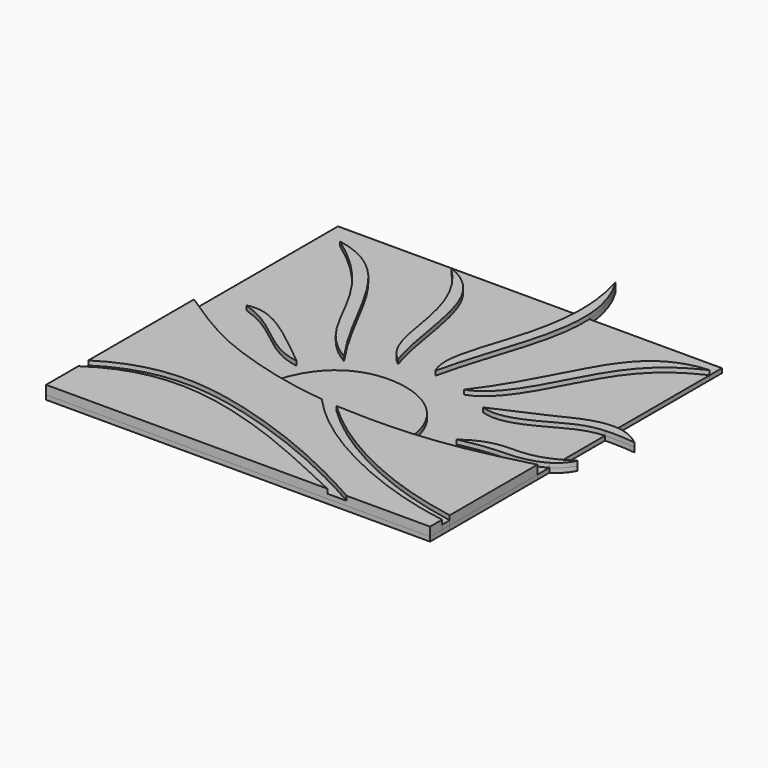
from build123d import *

# Parameters (mm, degrees)
F1_DEPTH = 0.8
F2_DEPTH = 0.8
F4_DEPTH = 0.8


# Not quite as in the source:
# - the dataset's text gives a spline's control points without its knots; the knots are read off the source's solid


with BuildPart() as f1:
    # F0 (on Top) → F1 (new body)
    with BuildSketch(Plane.XY):
        with BuildLine():
            Line((34.9730342203, 35.0006110966), (10.9699166685, 35.0006110966))
            add(Edge.make_bspline(
                [(10.9699166685, 35.0006110966), (11.4434143594, 26.4683997801), (6.9927337903, 17.8281453772), (4.7980677336, 7.8657846898)],
                knots=[10.4639255088, 10.4639255088, 10.4639255088, 10.4639255088, 37.2667273863, 37.2667273863, 37.2667273863, 37.2667273863], degree=3))
            add(Edge.make_bspline(
                [(9.1649998173, 35.0006110966), (8.9947581749, 22.5710061914), (1.9450564413, 13.7213998068), (4.7980677336, 7.8657846898)],
                knots=[7.4607386128, 7.4607386128, 7.4607386128, 7.4607386128, 37.2667273863, 37.2667273863, 37.2667273863, 37.2667273863], degree=3))
            Line((9.1649998173, 35.0006110966), (-34.5254550172, 35.0006110966))
            Line((-34.5254550172, 35.0006110966), (-34.5254550172, 2.4173662354))
            add(Edge.make_bspline(
                [(-34.5254550172, 2.4173662354), (-27.0376804173, -2.6116999925), (-21.9956358256, -5.211225175), (-13.8138692011, -7.7319000425), (-11.0227311637, -8.421960214)],
                knots=[0, 0, 0, 0, 0.5006994626, 0.7376571396, 0.7376571396, 0.7376571396, 0.7376571396], degree=3))
            add(Edge.make_bspline(
                [(-11.0227311637, -8.421960214), (-8.8453157151, -0.8208052436), (1.8576873576, 4.9563290965), (14.2170952187, -2.2695153177), (14.8043119806, -10.429123426)],
                knots=[0, 0, 0, 0, 0.4927942215, 1, 1, 1, 1], degree=3))
            add(Edge.make_bspline(
                [(14.8043119806, -10.429123426), (16.5213615363, -10.3106762034), (23.4560587989, -9.6183687732), (30.1043070095, -8.0231877273), (34.9773075939, -6.7529535132)],
                knots=[0.3679463332, 0.3679463332, 0.3679463332, 0.3679463332, 0.5212374468, 1, 1, 1, 1], degree=3))
            Line((34.9773075939, -6.7529535132), (34.9770299958, -4.040644467))
            add(Edge.make_bspline(
                [(20.261824131, -6.674728822), (25.9323026985, -5.3960913792), (28.2483273712, -6.1310401757), (33.4074649083, -4.9876865132), (34.9770299958, -4.040644467)],
                knots=[0, 0, 0, 0, 0.514073902, 0.7971639338, 0.7971639338, 0.7971639338, 0.7971639338], degree=3))
            add(Edge.make_bspline(
                [(20.261824131, -6.674728822), (24.2642636854, -3.7840772049), (28.8724834606, -4.3450209461), (32.8278065722, -3.6447079653), (34.976883526, -2.609541392)],
                knots=[0, 0, 0, 0, 0.5118221944, 0.8647946005, 0.8647946005, 0.8647946005, 0.8647946005], degree=3))
            Line((34.976883526, -2.609541392), (34.9757434519, 8.5297036957))
            add(Edge.make_bspline(
                [(17.0930270106, 3.331998596), (21.0957173258, 1.9421754405), (28.3670720206, 6.719546536), (32.5488536668, 8.3655302085), (34.9757434519, 8.5297036957)],
                knots=[0, 0, 0, 0, 0.5070444455, 0.8166137967, 0.8166137967, 0.8166137967, 0.8166137967], degree=3))
            add(Edge.make_bspline(
                [(17.0930270106, 3.331998596), (24.4312938303, 6.6675744019), (25.142738508, 6.7759703545), (32.0404376887, 10.3392415102), (34.9755569111, 10.3523255806)],
                knots=[0, 0, 0, 0, 0.4853131484, 0.8039573304, 0.8039573304, 0.8039573304, 0.8039573304], degree=3))
            Line((34.9755569111, 10.3523255806), (34.9733161214, 32.246258361))
            Line((34.9733161214, 32.246258361), (34.9730342203, 35.0006110966))
        make_face()
        with BuildLine():
            add(Edge.make_bspline(
                [(-28.5548307002, 6.8228477612), (-21.2621595711, 4.5322012156), (-18.9715120941, -1.030798303), (-12.3800588772, -2.0125040319)],
                knots=[0, 0, 0, 0, 18.4305910061, 18.4305910061, 18.4305910061, 18.4305910061], degree=3))
            add(Edge.make_bspline(
                [(-28.5548307002, 6.8228477612), (-24.1137798876, 8.0850413069), (-18.9715120941, 3.1765124295), (-12.3800588772, -2.0125040319)],
                knots=[0, 0, 0, 0, 18.4305910061, 18.4305910061, 18.4305910061, 18.4305910061], degree=3))
        make_face(mode=Mode.SUBTRACT)
        with BuildLine():
            add(Edge.make_bspline(
                [(-30.4424781352, 30.3799584508), (-14.8932319134, 19.365908578), (-18.1915573776, 9.1764414683), (-8.0609880388, 3.2865752)],
                knots=[0, 0, 0, 0, 35.1423180071, 35.1423180071, 35.1423180071, 35.1423180071], degree=3))
            add(Edge.make_bspline(
                [(-30.4424781352, 30.3799584508), (-18.3093566447, 28.1418096274), (-16.7779885232, 15.8319901675), (-8.0609880388, 3.2865752)],
                knots=[0, 0, 0, 0, 35.1423180071, 35.1423180071, 35.1423180071, 35.1423180071], degree=3))
        make_face(mode=Mode.SUBTRACT)
        with BuildLine():
            add(Edge.make_bspline(
                [(-13.0653008819, 33.8075049222), (-3.1436614227, 24.1144448519), (-7.886134088, 12.1958628297), (-1.5212370781, 7.3285889812)],
                knots=[0, 0, 0, 0, 28.885955039, 28.885955039, 28.885955039, 28.885955039], degree=3))
            add(Edge.make_bspline(
                [(-13.0653008819, 33.8075049222), (-3.081260249, 29.9177337438), (-5.0780908205, 18.31115596), (-1.5212370781, 7.3285889812)],
                knots=[0, 0, 0, 0, 28.885955039, 28.885955039, 28.885955039, 28.885955039], degree=3))
        make_face(mode=Mode.SUBTRACT)
        with BuildLine():
            add(Edge.make_bspline(
                [(34.9733161214, 32.246258361), (26.694862172, 31.7585282028), (20.0014700507, 20.5728578228), (15.3970348817, 10.8755724271), (11.565268971, 5.9131206945)],
                knots=[0, 0, 0, 0, 0.5086442243, 1, 1, 1, 1], degree=3))
            add(Edge.make_bspline(
                [(34.9733161214, 32.246258361), (28.0495304614, 29.0197413415), (22.3665736308, 20.9948728696), (16.2112628167, 7.3571462772), (11.565268971, 5.9131206945)],
                knots=[0, 0, 0, 0, 0.5063383757, 1, 1, 1, 1], degree=3))
        make_face(mode=Mode.SUBTRACT)
        with BuildLine():
            add(Edge.make_bspline(
                [(-34.5254550172, 2.4173662354), (-27.0376804173, -2.6116999925), (-21.9956358256, -5.211225175), (-13.8138692011, -7.7319000425), (-11.0227311637, -8.421960214)],
                knots=[0, 0, 0, 0, 0.5006994626, 0.7376571396, 0.7376571396, 0.7376571396, 0.7376571396], degree=3))
            Line((-34.5254550172, 2.4173662354), (-34.5254550172, -21.5029727188))
            add(Edge.make_bspline(
                [(-34.5254550172, -21.5029727188), (-25.4725657698, -15.6213664106), (-6.7297761633, -18.0960890657), (10.8723963711, -25.9276739276), (19.8863351902, -31.0484187179)],
                knots=[0, 0, 0, 0, 0.4889236203, 1, 1, 1, 1], degree=3))
            Line((19.8863351902, -31.0484187179), (34.9797941745, -31.0484187179))
            Line((34.9797941745, -31.0484187179), (34.9795152363, -28.32301612))
            add(Edge.make_bspline(
                [(-1.3718163174, -10.1225785816), (3.8546116383, -15.8494096152), (16.1560983213, -23.3323485383), (28.3092996314, -27.2113128984), (34.9795152363, -28.32301612)],
                knots=[0, 0, 0, 0, 0.5146424098, 1, 1, 1, 1], degree=3))
            add(Edge.make_bspline(
                [(-11.0227311637, -8.421960214), (-7.9325795984, -9.1859462621), (-4.6427454411, -9.8032650716), (-1.3718163174, -10.1225785816)],
                knots=[0.7376571396, 0.7376571396, 0.7376571396, 0.7376571396, 1, 1, 1, 1], degree=3))
        make_face()
        with BuildLine():
            add(Edge.make_bspline(
                [(-34.5254550172, -23.7555388327), (-26.0445526205, -17.8952354176), (-8.0264611969, -19.3880719353), (8.0517873689, -27.1572651783), (16.3802922747, -31.0484187179)],
                knots=[0, 0, 0, 0, 0.4951755821, 1, 1, 1, 1], degree=3))
            Line((-34.5254550172, -23.7555388327), (-34.5254550172, -31.0484187179))
            Line((-34.5254550172, -31.0484187179), (16.3802922747, -31.0484187179))
        make_face()
        with BuildLine():
            add(Edge.make_bspline(
                [(14.8043119806, -10.429123426), (16.5213615363, -10.3106762034), (23.4560587989, -9.6183687732), (30.1043070095, -8.0231877273), (34.9773075939, -6.7529535132)],
                knots=[0.3679463332, 0.3679463332, 0.3679463332, 0.3679463332, 0.5212374468, 1, 1, 1, 1], degree=3))
            add(Edge.make_bspline(
                [(1.5781647526, -10.4776900262), (6.3586774053, -10.7127967269), (10.6828591895, -10.7134335873), (14.8043119806, -10.429123426)],
                knots=[0, 0, 0, 0, 0.3679463332, 0.3679463332, 0.3679463332, 0.3679463332], degree=3))
            add(Edge.make_bspline(
                [(1.5781647526, -10.4776900262), (6.0786014384, -14.8114432857), (16.8554999855, -21.6973110945), (28.304374887, -25.3758922346), (34.9793388523, -26.599633516)],
                knots=[0, 0, 0, 0, 0.4979262009, 1, 1, 1, 1], degree=3))
            Line((34.9793388523, -26.599633516), (34.9773075939, -6.7529535132))
        make_face()
        with BuildLine():
            add(Edge.make_bspline(
                [(-11.0227311637, -8.421960214), (-8.8453157151, -0.8208052436), (1.8576873576, 4.9563290965), (14.2170952187, -2.2695153177), (14.8043119806, -10.429123426)],
                knots=[0, 0, 0, 0, 0.4927942215, 1, 1, 1, 1], degree=3))
            add(Edge.make_bspline(
                [(-11.0227311637, -8.421960214), (-7.9325795984, -9.1859462621), (-4.6427454411, -9.8032650716), (-1.3718163174, -10.1225785816)],
                knots=[0.7376571396, 0.7376571396, 0.7376571396, 0.7376571396, 1, 1, 1, 1], degree=3))
            add(Edge.make_bspline(
                [(-1.3718163174, -10.1225785816), (3.8546116383, -15.8494096152), (16.1560983213, -23.3323485383), (28.3092996314, -27.2113128984), (34.9795152363, -28.32301612)],
                knots=[0, 0, 0, 0, 0.5146424098, 1, 1, 1, 1], degree=3))
            Line((34.9795152363, -28.32301612), (34.9793388523, -26.599633516))
            add(Edge.make_bspline(
                [(1.5781647526, -10.4776900262), (6.0786014384, -14.8114432857), (16.8554999855, -21.6973110945), (28.304374887, -25.3758922346), (34.9793388523, -26.599633516)],
                knots=[0, 0, 0, 0, 0.4979262009, 1, 1, 1, 1], degree=3))
            add(Edge.make_bspline(
                [(1.5781647526, -10.4776900262), (6.3586774053, -10.7127967269), (10.6828591895, -10.7134335873), (14.8043119806, -10.429123426)],
                knots=[0, 0, 0, 0, 0.3679463332, 0.3679463332, 0.3679463332, 0.3679463332], degree=3))
        make_face()
        with BuildLine():
            add(Edge.make_bspline(
                [(-34.5254550172, -21.5029727188), (-25.4725657698, -15.6213664106), (-6.7297761633, -18.0960890657), (10.8723963711, -25.9276739276), (19.8863351902, -31.0484187179)],
                knots=[0, 0, 0, 0, 0.4889236203, 1, 1, 1, 1], degree=3))
            Line((-34.5254550172, -21.5029727188), (-34.5254550172, -23.7555388327))
            add(Edge.make_bspline(
                [(-34.5254550172, -23.7555388327), (-26.0445526205, -17.8952354176), (-8.0264611969, -19.3880719353), (8.0517873689, -27.1572651783), (16.3802922747, -31.0484187179)],
                knots=[0, 0, 0, 0, 0.4951755821, 1, 1, 1, 1], degree=3))
            Line((16.3802922747, -31.0484187179), (19.8863351902, -31.0484187179))
        make_face()
        with BuildLine():
            add(Edge.make_bspline(
                [(-30.4424781352, 30.3799584508), (-18.3093566447, 28.1418096274), (-16.7779885232, 15.8319901675), (-8.0609880388, 3.2865752)],
                knots=[0, 0, 0, 0, 35.1423180071, 35.1423180071, 35.1423180071, 35.1423180071], degree=3))
            add(Edge.make_bspline(
                [(-30.4424781352, 30.3799584508), (-14.8932319134, 19.365908578), (-18.1915573776, 9.1764414683), (-8.0609880388, 3.2865752)],
                knots=[0, 0, 0, 0, 35.1423180071, 35.1423180071, 35.1423180071, 35.1423180071], degree=3))
        make_face()
        with BuildLine():
            add(Edge.make_bspline(
                [(34.9733161214, 32.246258361), (28.0495304614, 29.0197413415), (22.3665736308, 20.9948728696), (16.2112628167, 7.3571462772), (11.565268971, 5.9131206945)],
                knots=[0, 0, 0, 0, 0.5063383757, 1, 1, 1, 1], degree=3))
            add(Edge.make_bspline(
                [(34.9733161214, 32.246258361), (26.694862172, 31.7585282028), (20.0014700507, 20.5728578228), (15.3970348817, 10.8755724271), (11.565268971, 5.9131206945)],
                knots=[0, 0, 0, 0, 0.5086442243, 1, 1, 1, 1], degree=3))
        make_face()
        with BuildLine():
            add(Edge.make_bspline(
                [(7.7365408652, 45.0164824724), (9.8496850647, 41.6461653484), (10.7850611974, 38.3316219383), (10.9699166685, 35.0006110966)],
                knots=[0, 0, 0, 0, 10.4639255088, 10.4639255088, 10.4639255088, 10.4639255088], degree=3))
            add(Edge.make_bspline(
                [(7.7365408652, 45.0164824724), (8.8191927924, 41.4474264531), (9.2076130117, 38.1118661522), (9.1649998173, 35.0006110966)],
                knots=[0, 0, 0, 0, 7.4607386128, 7.4607386128, 7.4607386128, 7.4607386128], degree=3))
            add(Edge.make_bspline(
                [(9.1649998173, 35.0006110966), (8.9947581749, 22.5710061914), (1.9450564413, 13.7213998068), (4.7980677336, 7.8657846898)],
                knots=[7.4607386128, 7.4607386128, 7.4607386128, 7.4607386128, 37.2667273863, 37.2667273863, 37.2667273863, 37.2667273863], degree=3))
            add(Edge.make_bspline(
                [(10.9699166685, 35.0006110966), (11.4434143594, 26.4683997801), (6.9927337903, 17.8281453772), (4.7980677336, 7.8657846898)],
                knots=[10.4639255088, 10.4639255088, 10.4639255088, 10.4639255088, 37.2667273863, 37.2667273863, 37.2667273863, 37.2667273863], degree=3))
        make_face()
        with BuildLine():
            add(Edge.make_bspline(
                [(-13.0653008819, 33.8075049222), (-3.081260249, 29.9177337438), (-5.0780908205, 18.31115596), (-1.5212370781, 7.3285889812)],
                knots=[0, 0, 0, 0, 28.885955039, 28.885955039, 28.885955039, 28.885955039], degree=3))
            add(Edge.make_bspline(
                [(-13.0653008819, 33.8075049222), (-3.1436614227, 24.1144448519), (-7.886134088, 12.1958628297), (-1.5212370781, 7.3285889812)],
                knots=[0, 0, 0, 0, 28.885955039, 28.885955039, 28.885955039, 28.885955039], degree=3))
        make_face()
        with BuildLine():
            add(Edge.make_bspline(
                [(34.9755569111, 10.3523255806), (36.7813598733, 10.3603754249), (38.6633412268, 9.8387998398), (40.4420569539, 8.3353621885)],
                knots=[0.8039573304, 0.8039573304, 0.8039573304, 0.8039573304, 1, 1, 1, 1], degree=3))
            add(Edge.make_bspline(
                [(17.0930270106, 3.331998596), (24.4312938303, 6.6675744019), (25.142738508, 6.7759703545), (32.0404376887, 10.3392415102), (34.9755569111, 10.3523255806)],
                knots=[0, 0, 0, 0, 0.4853131484, 0.8039573304, 0.8039573304, 0.8039573304, 0.8039573304], degree=3))
            add(Edge.make_bspline(
                [(17.0930270106, 3.331998596), (21.0957173258, 1.9421754405), (28.3670720206, 6.719546536), (32.5488536668, 8.3655302085), (34.9757434519, 8.5297036957)],
                knots=[0, 0, 0, 0, 0.5070444455, 0.8166137967, 0.8166137967, 0.8166137967, 0.8166137967], degree=3))
            add(Edge.make_bspline(
                [(34.9757434519, 8.5297036957), (36.4134119483, 8.626958648), (38.1464287997, 8.5628568174), (40.4420569539, 8.3353621885)],
                knots=[0.8166137967, 0.8166137967, 0.8166137967, 0.8166137967, 1, 1, 1, 1], degree=3))
        make_face()
        with BuildLine():
            add(Edge.make_bspline(
                [(-28.5548307002, 6.8228477612), (-24.1137798876, 8.0850413069), (-18.9715120941, 3.1765124295), (-12.3800588772, -2.0125040319)],
                knots=[0, 0, 0, 0, 18.4305910061, 18.4305910061, 18.4305910061, 18.4305910061], degree=3))
            add(Edge.make_bspline(
                [(-28.5548307002, 6.8228477612), (-21.2621595711, 4.5322012156), (-18.9715120941, -1.030798303), (-12.3800588772, -2.0125040319)],
                knots=[0, 0, 0, 0, 18.4305910061, 18.4305910061, 18.4305910061, 18.4305910061], degree=3))
        make_face()
        with BuildLine():
            add(Edge.make_bspline(
                [(34.976883526, -2.609541392), (35.8000833093, -2.213022832), (36.7017347712, -1.7065584186), (37.7180017531, -1.0598427616)],
                knots=[0.8647946005, 0.8647946005, 0.8647946005, 0.8647946005, 1, 1, 1, 1], degree=3))
            add(Edge.make_bspline(
                [(20.261824131, -6.674728822), (24.2642636854, -3.7840772049), (28.8724834606, -4.3450209461), (32.8278065722, -3.6447079653), (34.976883526, -2.609541392)],
                knots=[0, 0, 0, 0, 0.5118221944, 0.8647946005, 0.8647946005, 0.8647946005, 0.8647946005], degree=3))
            add(Edge.make_bspline(
                [(20.261824131, -6.674728822), (25.9323026985, -5.3960913792), (28.2483273712, -6.1310401757), (33.4074649083, -4.9876865132), (34.9770299958, -4.040644467)],
                knots=[0, 0, 0, 0, 0.514073902, 0.7971639338, 0.7971639338, 0.7971639338, 0.7971639338], degree=3))
            add(Edge.make_bspline(
                [(34.9770299958, -4.040644467), (36.1016347939, -3.3620819546), (37.0914481775, -2.4057729455), (37.7180017531, -1.0598427616)],
                knots=[0.7971639338, 0.7971639338, 0.7971639338, 0.7971639338, 1, 1, 1, 1], degree=3))
        make_face()
    extrude(amount=-F1_DEPTH)


with BuildPart() as f2:
    # F0 (on Top) → F2 (new body)
    with BuildSketch(Plane.XY):
        with BuildLine():
            add(Edge.make_bspline(
                [(-28.5548307002, 6.8228477612), (-24.1137798876, 8.0850413069), (-18.9715120941, 3.1765124295), (-12.3800588772, -2.0125040319)],
                knots=[0, 0, 0, 0, 18.4305910061, 18.4305910061, 18.4305910061, 18.4305910061], degree=3))
            add(Edge.make_bspline(
                [(-28.5548307002, 6.8228477612), (-21.2621595711, 4.5322012156), (-18.9715120941, -1.030798303), (-12.3800588772, -2.0125040319)],
                knots=[0, 0, 0, 0, 18.4305910061, 18.4305910061, 18.4305910061, 18.4305910061], degree=3))
        make_face()
    extrude(amount=F2_DEPTH)


with BuildPart() as f2b:
    # F0 (on Top) → F2, piece 2 (new body)
    with BuildSketch(Plane.XY):
        with BuildLine():
            add(Edge.make_bspline(
                [(-30.4424781352, 30.3799584508), (-18.3093566447, 28.1418096274), (-16.7779885232, 15.8319901675), (-8.0609880388, 3.2865752)],
                knots=[0, 0, 0, 0, 35.1423180071, 35.1423180071, 35.1423180071, 35.1423180071], degree=3))
            add(Edge.make_bspline(
                [(-30.4424781352, 30.3799584508), (-14.8932319134, 19.365908578), (-18.1915573776, 9.1764414683), (-8.0609880388, 3.2865752)],
                knots=[0, 0, 0, 0, 35.1423180071, 35.1423180071, 35.1423180071, 35.1423180071], degree=3))
        make_face()
    extrude(amount=F2_DEPTH)


with BuildPart() as f2c:
    # F0 (on Top) → F2, piece 3 (new body)
    with BuildSketch(Plane.XY):
        with BuildLine():
            add(Edge.make_bspline(
                [(-13.0653008819, 33.8075049222), (-3.081260249, 29.9177337438), (-5.0780908205, 18.31115596), (-1.5212370781, 7.3285889812)],
                knots=[0, 0, 0, 0, 28.885955039, 28.885955039, 28.885955039, 28.885955039], degree=3))
            add(Edge.make_bspline(
                [(-13.0653008819, 33.8075049222), (-3.1436614227, 24.1144448519), (-7.886134088, 12.1958628297), (-1.5212370781, 7.3285889812)],
                knots=[0, 0, 0, 0, 28.885955039, 28.885955039, 28.885955039, 28.885955039], degree=3))
        make_face()
    extrude(amount=F2_DEPTH)


with BuildPart() as f2d:
    # F0 (on Top) → F2, piece 4 (new body)
    with BuildSketch(Plane.XY):
        with BuildLine():
            add(Edge.make_bspline(
                [(34.9733161214, 32.246258361), (28.0495304614, 29.0197413415), (22.3665736308, 20.9948728696), (16.2112628167, 7.3571462772), (11.565268971, 5.9131206945)],
                knots=[0, 0, 0, 0, 0.5063383757, 1, 1, 1, 1], degree=3))
            add(Edge.make_bspline(
                [(34.9733161214, 32.246258361), (26.694862172, 31.7585282028), (20.0014700507, 20.5728578228), (15.3970348817, 10.8755724271), (11.565268971, 5.9131206945)],
                knots=[0, 0, 0, 0, 0.5086442243, 1, 1, 1, 1], degree=3))
        make_face()
    extrude(amount=F2_DEPTH)


with BuildPart() as f2e:
    # F0 (on Top) → F2, piece 5 (new body)
    with BuildSketch(Plane.XY):
        with BuildLine():
            add(Edge.make_bspline(
                [(34.9755569111, 10.3523255806), (36.7813598733, 10.3603754249), (38.6633412268, 9.8387998398), (40.4420569539, 8.3353621885)],
                knots=[0.8039573304, 0.8039573304, 0.8039573304, 0.8039573304, 1, 1, 1, 1], degree=3))
            add(Edge.make_bspline(
                [(17.0930270106, 3.331998596), (24.4312938303, 6.6675744019), (25.142738508, 6.7759703545), (32.0404376887, 10.3392415102), (34.9755569111, 10.3523255806)],
                knots=[0, 0, 0, 0, 0.4853131484, 0.8039573304, 0.8039573304, 0.8039573304, 0.8039573304], degree=3))
            add(Edge.make_bspline(
                [(17.0930270106, 3.331998596), (21.0957173258, 1.9421754405), (28.3670720206, 6.719546536), (32.5488536668, 8.3655302085), (34.9757434519, 8.5297036957)],
                knots=[0, 0, 0, 0, 0.5070444455, 0.8166137967, 0.8166137967, 0.8166137967, 0.8166137967], degree=3))
            add(Edge.make_bspline(
                [(34.9757434519, 8.5297036957), (36.4134119483, 8.626958648), (38.1464287997, 8.5628568174), (40.4420569539, 8.3353621885)],
                knots=[0.8166137967, 0.8166137967, 0.8166137967, 0.8166137967, 1, 1, 1, 1], degree=3))
        make_face()
    extrude(amount=F2_DEPTH)


with BuildPart() as f2f:
    # F0 (on Top) → F2, piece 6 (new body)
    with BuildSketch(Plane.XY):
        with BuildLine():
            add(Edge.make_bspline(
                [(7.7365408652, 45.0164824724), (9.8496850647, 41.6461653484), (10.7850611974, 38.3316219383), (10.9699166685, 35.0006110966)],
                knots=[0, 0, 0, 0, 10.4639255088, 10.4639255088, 10.4639255088, 10.4639255088], degree=3))
            add(Edge.make_bspline(
                [(7.7365408652, 45.0164824724), (8.8191927924, 41.4474264531), (9.2076130117, 38.1118661522), (9.1649998173, 35.0006110966)],
                knots=[0, 0, 0, 0, 7.4607386128, 7.4607386128, 7.4607386128, 7.4607386128], degree=3))
            add(Edge.make_bspline(
                [(9.1649998173, 35.0006110966), (8.9947581749, 22.5710061914), (1.9450564413, 13.7213998068), (4.7980677336, 7.8657846898)],
                knots=[7.4607386128, 7.4607386128, 7.4607386128, 7.4607386128, 37.2667273863, 37.2667273863, 37.2667273863, 37.2667273863], degree=3))
            add(Edge.make_bspline(
                [(10.9699166685, 35.0006110966), (11.4434143594, 26.4683997801), (6.9927337903, 17.8281453772), (4.7980677336, 7.8657846898)],
                knots=[10.4639255088, 10.4639255088, 10.4639255088, 10.4639255088, 37.2667273863, 37.2667273863, 37.2667273863, 37.2667273863], degree=3))
        make_face()
    extrude(amount=F2_DEPTH)


with BuildPart() as f2g:
    # F0 (on Top) → F2, piece 7 (new body)
    with BuildSketch(Plane.XY):
        with BuildLine():
            add(Edge.make_bspline(
                [(34.976883526, -2.609541392), (35.8000833093, -2.213022832), (36.7017347712, -1.7065584186), (37.7180017531, -1.0598427616)],
                knots=[0.8647946005, 0.8647946005, 0.8647946005, 0.8647946005, 1, 1, 1, 1], degree=3))
            add(Edge.make_bspline(
                [(20.261824131, -6.674728822), (24.2642636854, -3.7840772049), (28.8724834606, -4.3450209461), (32.8278065722, -3.6447079653), (34.976883526, -2.609541392)],
                knots=[0, 0, 0, 0, 0.5118221944, 0.8647946005, 0.8647946005, 0.8647946005, 0.8647946005], degree=3))
            add(Edge.make_bspline(
                [(20.261824131, -6.674728822), (25.9323026985, -5.3960913792), (28.2483273712, -6.1310401757), (33.4074649083, -4.9876865132), (34.9770299958, -4.040644467)],
                knots=[0, 0, 0, 0, 0.514073902, 0.7971639338, 0.7971639338, 0.7971639338, 0.7971639338], degree=3))
            add(Edge.make_bspline(
                [(34.9770299958, -4.040644467), (36.1016347939, -3.3620819546), (37.0914481775, -2.4057729455), (37.7180017531, -1.0598427616)],
                knots=[0.7971639338, 0.7971639338, 0.7971639338, 0.7971639338, 1, 1, 1, 1], degree=3))
        make_face()
    extrude(amount=F2_DEPTH)


with BuildPart() as f2h:
    # F0 (on Top) → F2, piece 8 (new body)
    with BuildSketch(Plane.XY):
        with BuildLine():
            add(Edge.make_bspline(
                [(-11.0227311637, -8.421960214), (-8.8453157151, -0.8208052436), (1.8576873576, 4.9563290965), (14.2170952187, -2.2695153177), (14.8043119806, -10.429123426)],
                knots=[0, 0, 0, 0, 0.4927942215, 1, 1, 1, 1], degree=3))
            add(Edge.make_bspline(
                [(-11.0227311637, -8.421960214), (-7.9325795984, -9.1859462621), (-4.6427454411, -9.8032650716), (-1.3718163174, -10.1225785816)],
                knots=[0.7376571396, 0.7376571396, 0.7376571396, 0.7376571396, 1, 1, 1, 1], degree=3))
            add(Edge.make_bspline(
                [(-1.3718163174, -10.1225785816), (3.8546116383, -15.8494096152), (16.1560983213, -23.3323485383), (28.3092996314, -27.2113128984), (34.9795152363, -28.32301612)],
                knots=[0, 0, 0, 0, 0.5146424098, 1, 1, 1, 1], degree=3))
            Line((34.9795152363, -28.32301612), (34.9793388523, -26.599633516))
            add(Edge.make_bspline(
                [(1.5781647526, -10.4776900262), (6.0786014384, -14.8114432857), (16.8554999855, -21.6973110945), (28.304374887, -25.3758922346), (34.9793388523, -26.599633516)],
                knots=[0, 0, 0, 0, 0.4979262009, 1, 1, 1, 1], degree=3))
            add(Edge.make_bspline(
                [(1.5781647526, -10.4776900262), (6.3586774053, -10.7127967269), (10.6828591895, -10.7134335873), (14.8043119806, -10.429123426)],
                knots=[0, 0, 0, 0, 0.3679463332, 0.3679463332, 0.3679463332, 0.3679463332], degree=3))
        make_face()
        with BuildLine():
            add(Edge.make_bspline(
                [(-34.5254550172, -21.5029727188), (-25.4725657698, -15.6213664106), (-6.7297761633, -18.0960890657), (10.8723963711, -25.9276739276), (19.8863351902, -31.0484187179)],
                knots=[0, 0, 0, 0, 0.4889236203, 1, 1, 1, 1], degree=3))
            Line((-34.5254550172, -21.5029727188), (-34.5254550172, -23.7555388327))
            add(Edge.make_bspline(
                [(-34.5254550172, -23.7555388327), (-26.0445526205, -17.8952354176), (-8.0264611969, -19.3880719353), (8.0517873689, -27.1572651783), (16.3802922747, -31.0484187179)],
                knots=[0, 0, 0, 0, 0.4951755821, 1, 1, 1, 1], degree=3))
            Line((16.3802922747, -31.0484187179), (19.8863351902, -31.0484187179))
        make_face()
        with BuildLine():
            add(Edge.make_bspline(
                [(-34.5254550172, 2.4173662354), (-27.0376804173, -2.6116999925), (-21.9956358256, -5.211225175), (-13.8138692011, -7.7319000425), (-11.0227311637, -8.421960214)],
                knots=[0, 0, 0, 0, 0.5006994626, 0.7376571396, 0.7376571396, 0.7376571396, 0.7376571396], degree=3))
            Line((-34.5254550172, 2.4173662354), (-34.5254550172, -21.5029727188))
            add(Edge.make_bspline(
                [(-34.5254550172, -21.5029727188), (-25.4725657698, -15.6213664106), (-6.7297761633, -18.0960890657), (10.8723963711, -25.9276739276), (19.8863351902, -31.0484187179)],
                knots=[0, 0, 0, 0, 0.4889236203, 1, 1, 1, 1], degree=3))
            Line((19.8863351902, -31.0484187179), (34.9797941745, -31.0484187179))
            Line((34.9797941745, -31.0484187179), (34.9795152363, -28.32301612))
            add(Edge.make_bspline(
                [(-1.3718163174, -10.1225785816), (3.8546116383, -15.8494096152), (16.1560983213, -23.3323485383), (28.3092996314, -27.2113128984), (34.9795152363, -28.32301612)],
                knots=[0, 0, 0, 0, 0.5146424098, 1, 1, 1, 1], degree=3))
            add(Edge.make_bspline(
                [(-11.0227311637, -8.421960214), (-7.9325795984, -9.1859462621), (-4.6427454411, -9.8032650716), (-1.3718163174, -10.1225785816)],
                knots=[0.7376571396, 0.7376571396, 0.7376571396, 0.7376571396, 1, 1, 1, 1], degree=3))
        make_face()
        with BuildLine():
            add(Edge.make_bspline(
                [(-34.5254550172, -23.7555388327), (-26.0445526205, -17.8952354176), (-8.0264611969, -19.3880719353), (8.0517873689, -27.1572651783), (16.3802922747, -31.0484187179)],
                knots=[0, 0, 0, 0, 0.4951755821, 1, 1, 1, 1], degree=3))
            Line((-34.5254550172, -23.7555388327), (-34.5254550172, -31.0484187179))
            Line((-34.5254550172, -31.0484187179), (16.3802922747, -31.0484187179))
        make_face()
        with BuildLine():
            add(Edge.make_bspline(
                [(14.8043119806, -10.429123426), (16.5213615363, -10.3106762034), (23.4560587989, -9.6183687732), (30.1043070095, -8.0231877273), (34.9773075939, -6.7529535132)],
                knots=[0.3679463332, 0.3679463332, 0.3679463332, 0.3679463332, 0.5212374468, 1, 1, 1, 1], degree=3))
            add(Edge.make_bspline(
                [(1.5781647526, -10.4776900262), (6.3586774053, -10.7127967269), (10.6828591895, -10.7134335873), (14.8043119806, -10.429123426)],
                knots=[0, 0, 0, 0, 0.3679463332, 0.3679463332, 0.3679463332, 0.3679463332], degree=3))
            add(Edge.make_bspline(
                [(1.5781647526, -10.4776900262), (6.0786014384, -14.8114432857), (16.8554999855, -21.6973110945), (28.304374887, -25.3758922346), (34.9793388523, -26.599633516)],
                knots=[0, 0, 0, 0, 0.4979262009, 1, 1, 1, 1], degree=3))
            Line((34.9793388523, -26.599633516), (34.9773075939, -6.7529535132))
        make_face()
    extrude(amount=F2_DEPTH)

    # F3 (on face) → F4 (join)
    with BuildSketch(Plane.XY.offset(0.8)):
        with BuildLine():
            add(Edge.make_bspline(
                [(-34.5254550172, -23.7555388327), (-26.0445526205, -17.8952354176), (-8.0264611969, -19.3880719353), (8.0517873689, -27.1572651783), (16.3802922747, -31.0484187179)],
                knots=[0, 0, 0, 0, 0.4951755821, 1, 1, 1, 1], degree=3))
            Line((-34.5254550172, -23.7555388327), (-34.5254550172, -31.0484187179))
            Line((-34.5254550172, -31.0484187179), (16.3802922747, -31.0484187179))
        make_face()
        with BuildLine():
            add(Edge.make_bspline(
                [(-34.5254550172, 2.4173662354), (-27.0376804173, -2.6116999925), (-21.9956358256, -5.211225175), (-13.8138692011, -7.7319000425), (-11.0227311637, -8.421960214)],
                knots=[0, 0, 0, 0, 0.5006994626, 0.7376571396, 0.7376571396, 0.7376571396, 0.7376571396], degree=3))
            Line((-34.5254550172, 2.4173662354), (-34.5254550172, -21.5029727188))
            add(Edge.make_bspline(
                [(-34.5254550172, -21.5029727188), (-25.4725657698, -15.6213664106), (-6.7297761633, -18.0960890657), (10.8723963711, -25.9276739276), (19.8863351902, -31.0484187179)],
                knots=[0, 0, 0, 0, 0.4889236203, 1, 1, 1, 1], degree=3))
            Line((19.8863351902, -31.0484187179), (34.9797941745, -31.0484187179))
            Line((34.9797941745, -31.0484187179), (34.9795152363, -28.32301612))
            add(Edge.make_bspline(
                [(-1.3718163174, -10.1225785816), (3.8546116383, -15.8494096152), (16.1560983213, -23.3323485383), (28.3092996314, -27.2113128984), (34.9795152363, -28.32301612)],
                knots=[0, 0, 0, 0, 0.5146424098, 1, 1, 1, 1], degree=3))
            add(Edge.make_bspline(
                [(-11.0227311637, -8.421960214), (-7.9325795984, -9.1859462621), (-4.6427454411, -9.8032650716), (-1.3718163174, -10.1225785816)],
                knots=[0.7376571396, 0.7376571396, 0.7376571396, 0.7376571396, 1, 1, 1, 1], degree=3))
        make_face()
        with BuildLine():
            add(Edge.make_bspline(
                [(14.8043119806, -10.429123426), (16.5213615363, -10.3106762034), (23.4560587989, -9.6183687732), (30.1043070095, -8.0231877273), (34.9773075939, -6.7529535132)],
                knots=[0.3679463332, 0.3679463332, 0.3679463332, 0.3679463332, 0.5212374468, 1, 1, 1, 1], degree=3))
            add(Edge.make_bspline(
                [(1.5781647526, -10.4776900262), (6.3586774053, -10.7127967269), (10.6828591895, -10.7134335873), (14.8043119806, -10.429123426)],
                knots=[0, 0, 0, 0, 0.3679463332, 0.3679463332, 0.3679463332, 0.3679463332], degree=3))
            add(Edge.make_bspline(
                [(1.5781647526, -10.4776900262), (6.0786014384, -14.8114432857), (16.8554999855, -21.6973110945), (28.304374887, -25.3758922346), (34.9793388523, -26.599633516)],
                knots=[0, 0, 0, 0, 0.4979262009, 1, 1, 1, 1], degree=3))
            Line((34.9793388523, -26.599633516), (34.9773075939, -6.7529535132))
        make_face()
    extrude(amount=F4_DEPTH)


solid = Compound([f1.part, f2.part, f2b.part, f2c.part, f2d.part, f2e.part, f2f.part, f2g.part, f2h.part])
